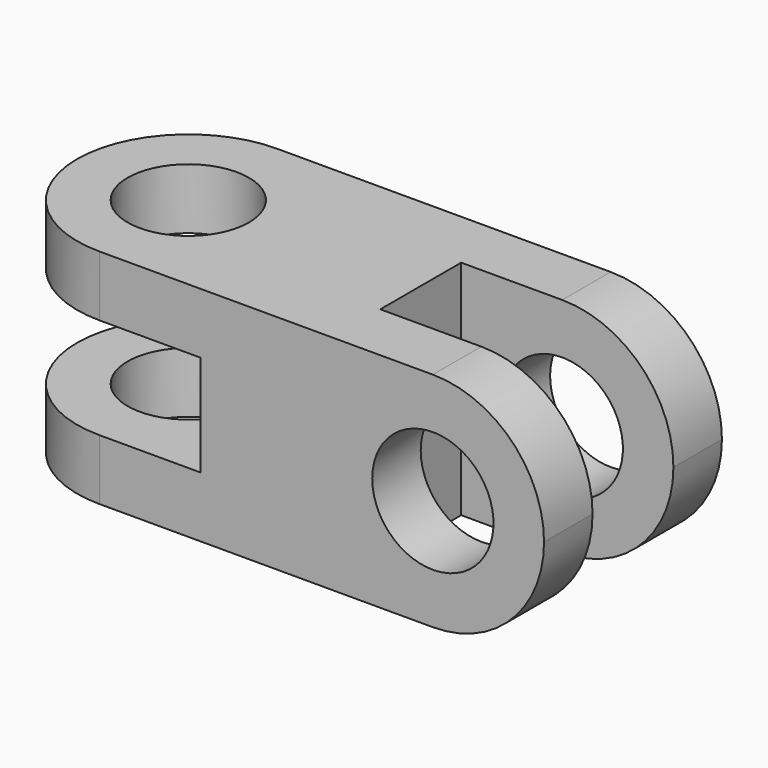
from build123d import *

# Parameters (mm, degrees)
F0_W      = 139.7
F0_H      = 55.88
F1_DEPTH  = 55.88
F2_W      = 101.6
F2_H      = 25.4
F3_DEPTH  = 55.881
F4_R      = 27.93999
F5_R      = 15.24
F6_DEPTH  = 55.881
F7_W      = 76.2
F7_H      = 25.4
F8_DEPTH  = 55.881
F9_R      = 15.24
F10_DEPTH = 55.881


# Not quite as in the source:
# - a fillet or chamfer is up to 0.001 mm smaller than in the source, because OpenCascade refuses the exact size


with BuildPart() as f1:
    # F0 (on Top) → F1 (new body)
    with BuildSketch(Plane.XY):
        with Locations((69.85, 27.94)):
            Rectangle(F0_W, F0_H)
    extrude(amount=F1_DEPTH)

    # F2 (on face) → F3 (cut, through all)
    with BuildSketch(Plane(origin=(0, 0, 0), x_dir=(1, 0, 0), z_dir=(0, 0, -1))):
        with Locations((137.16, -27.94)):
            Rectangle(F2_W, F2_H)
    extrude(amount=-F3_DEPTH, mode=Mode.SUBTRACT)

    # F4 (radius 27.94 in the source; OpenCascade refuses exactly that, so slightly less here)
    f4_edges = [f1.edges().sort_by_distance(p)[0] for p in [
        (139.7, 48.26, 55.88),
        (139.7, 7.62, 55.88),
        (139.7, 7.62, 0),
        (139.7, 48.26, 0),
        (0, 55.88, 27.94),
        (0, 0, 27.94),
    ]]
    fillet(f4_edges, radius=F4_R)

    # F5 (on face) → F6 (cut, through all)
    with BuildSketch(Plane(origin=(0, 55.88, 0), x_dir=(-1, 0, 0), z_dir=(0, 1, 0))):
        with Locations((-111.76, 27.94)):
            Circle(F5_R)
    extrude(amount=-F6_DEPTH, mode=Mode.SUBTRACT)

    # F7 (on face) → F8 (cut, through all)
    with BuildSketch(Plane(origin=(0, 55.88, 0), x_dir=(-1, 0, 0), z_dir=(0, 1, 0))):
        with Locations((-15.24, 27.94)):
            Rectangle(F7_W, F7_H)
    extrude(amount=-F8_DEPTH, mode=Mode.SUBTRACT)

    # F9 (on face) → F10 (cut, through all)
    with BuildSketch(Plane(origin=(0, 0, 0), x_dir=(1, 0, 0), z_dir=(0, 0, -1))):
        with Locations((27.94, -27.94)):
            Circle(F9_R)
    extrude(amount=-F10_DEPTH, mode=Mode.SUBTRACT)


solid = f1.part
